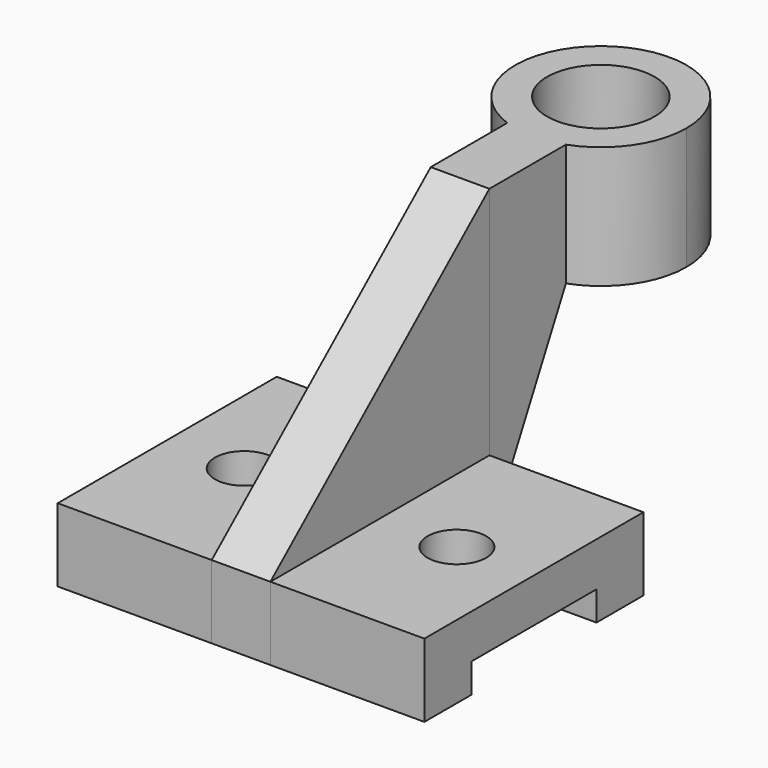
from build123d import *
from build123d import SkipClean  # not in build123d's __all__

# Parameters (mm, degrees)
F0_W      = 31.5
F0_H      = 56
F0_R      = 6
F1_DEPTH  = 15
F0_W_2    = 6
F2_DEPTH  = 63
F4_DEPTH  = 25
F5_W      = 12
F5_H      = 63
F6_DEPTH  = 36
F8_DEPTH  = 134.4
F9_DEPTH  = 25
F11_DEPTH = 25
F12_W     = 32
F12_H     = 6
F13_DEPTH = 101.3


# Not quite as in the source:
# - after a boolean that leaves OpenCascade's solid faulty, fix() repairs it


with BuildPart() as f1:
    # F0 (on Top) → F1 (new body)
    with BuildSketch(Plane.XY):
        with Locations((-21.75, 0)):
            Rectangle(F0_W, F0_H)
        with Locations((-21.75, 0)):
            Circle(F0_R, mode=Mode.SUBTRACT)
    extrude(amount=F1_DEPTH)


with BuildPart() as f1b:
    # F0 (on Top) → F1, piece 2 (new body)
    with BuildSketch(Plane.XY):
        with Locations((21.75, 0)):
            Rectangle(F0_W, F0_H)
        with Locations((21.75, 0)):
            Circle(F0_R, mode=Mode.SUBTRACT)
    extrude(amount=F1_DEPTH)


with BuildPart() as f2:
    # F0 (on Top) → F2 (new body)
    with BuildSketch(Plane.XY):
        with Locations((-3, 0)):
            Rectangle(F0_W_2, F0_H)
        with Locations((3, 0)):
            Rectangle(F0_W_2, F0_H)
    extrude(amount=F2_DEPTH)

    # F3 (on face) → F4 (cut)
    with BuildSketch(Plane.YZ.offset(6)):
        Polygon((-28, 63), (-28, 15), (28, 63), align=None)
    extrude(amount=-F4_DEPTH, mode=Mode.SUBTRACT)


with BuildPart() as f6:
    # F5 (on face) → F6 (new body)
    with BuildSketch(Plane(origin=(0, 28, 0), x_dir=(-1, 0, 0), z_dir=(0, 1, 0))):
        with Locations((0, 31.5)):
            Rectangle(F5_W, F5_H)
    extrude(amount=F6_DEPTH)

    # F7 (on face) → F8 (cut)
    with BuildSketch(Plane.XY.offset(63)):
        with BuildLine():
            Line((-6, 64), (-6, 54.7804555427))
            ThreePointArc((-6, 54.7804555427), (0, 53), (6, 54.7804555427))
            Line((6, 54.7804555427), (6, 64))
            Line((6, 64), (-6, 64))
        make_face()
    extrude(amount=-F8_DEPTH, mode=Mode.SUBTRACT)

    # F7 (on face) → F9 (join)
    with BuildSketch(Plane.XY.offset(63)):
        with BuildLine():
            ThreePointArc((-6, 54.7804555427), (-5.2440442409, 73.6695398029), (11, 64))
            ThreePointArc((11, 64), (9.6695398029, 58.7559557591), (6, 54.7804555427))
            Line((6, 54.7804555427), (6, 47.5607177772))
            ThreePointArc((6, 47.5607177772), (14.3396303997, 53.9687986761), (17.5, 64))
            ThreePointArc((17.5, 64), (-10.0312013239, 78.3396303997), (-6, 47.5607177772))
            Line((-6, 47.5607177772), (-6, 54.7804555427))
        make_face()
        with BuildLine():
            ThreePointArc((6, 54.7804555427), (0, 53), (-6, 54.7804555427))
            Line((-6, 54.7804555427), (-6, 47.5607177772))
            ThreePointArc((-6, 47.5607177772), (0, 46.5), (6, 47.5607177772))
            Line((6, 47.5607177772), (6, 54.7804555427))
        make_face()
        with BuildLine():
            ThreePointArc((6, 47.5607177772), (0, 46.5), (-6, 47.5607177772))
            Line((-6, 47.5607177772), (-6, 28))
            Line((-6, 28), (6, 28))
            Line((6, 28), (6, 47.5607177772))
        make_face()
    with SkipClean():  # cleaning this boolean's faces spoils the solid; the shape is the same uncleaned
        extrude(amount=-F9_DEPTH)

    # F10 (on face) → F11 (cut)
    with BuildSketch(Plane.YZ.offset(6)):
        Polygon((28, 0), (54.7804555427, 0), (54.7804555427, 38), (47.5607177772, 38), align=None)
    extrude(amount=-F11_DEPTH, mode=Mode.SUBTRACT)

    add(f6.part.fix(), mode=Mode.REPLACE)


with BuildPart() as f13_tool:
    # F12 (on face) → F13 (new body)
    with BuildSketch(Plane.YZ.offset(37.5)):
        with Locations((0, 3)):
            Rectangle(F12_W, F12_H)
    extrude(amount=-F13_DEPTH)


with BuildPart() as f1_1:
    add(f1.part, clean=False)

    # F13: cut by f13_tool
    add(f13_tool.part, mode=Mode.SUBTRACT)


with BuildPart() as f1b_1:
    add(f1b.part, clean=False)

    # F13: cut by f13_tool
    add(f13_tool.part, mode=Mode.SUBTRACT)


with BuildPart() as f2_1:
    add(f2.part, clean=False)

    # F13: cut by f13_tool
    add(f13_tool.part, mode=Mode.SUBTRACT)


solid = Compound([f6.part, f1_1.part, f1b_1.part, f2_1.part])
